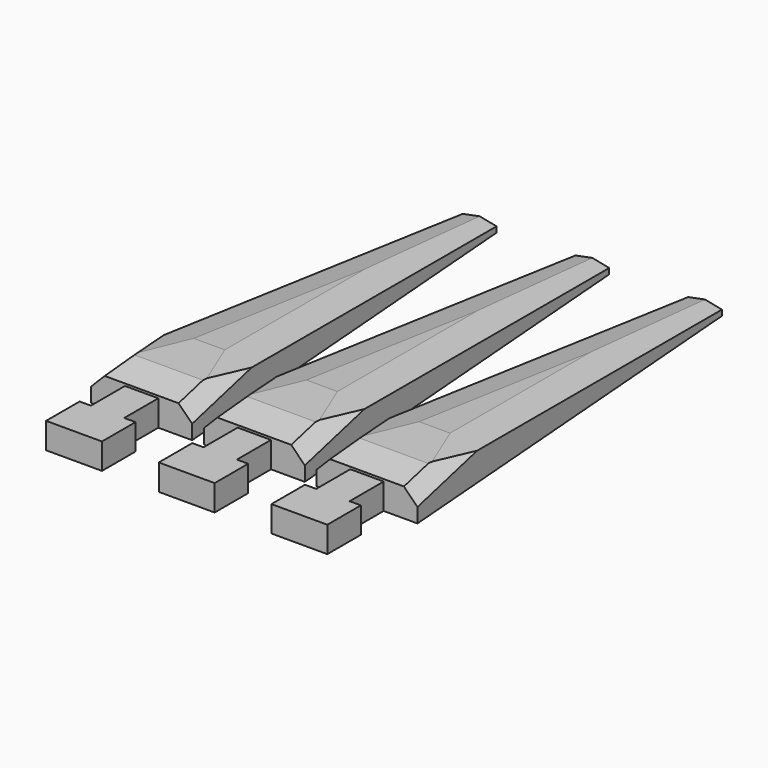
from build123d import *

# Parameters (mm, degrees)
F0_W        = 1.8796
F0_H        = 4.8006
F1_DEPTH    = 2.921
F2_DEPTH    = 3.81
F3_SIZE2    = 0.635
F3_SIZE     = 3.81
F4_SIZE2    = 2.54
F4_SIZE     = 38.1
F5_C1_SIZE  = 1.524
F5_C2_SIZE  = 1.524
F6_T1_DEPTH = 68.7483061083
F6_T3_DEPTH = 68.7483061083


# Not quite as in the source:
# - a fillet or chamfer that OpenCascade refuses, or shapes differently, is made with other operations: its cross-section is extruded or revolved along the edge and cut away or added


with BuildPart() as f1:
    # F0 (on Top) → F1 (new body)
    with BuildSketch(Plane.XY):
        Polygon((3.1496, -2.3622), (3.1496, 2.3622), (1.8796, 2.3622), (0, 2.3622), (-1.8796, 2.3622), (-3.1496, 2.3622), (-3.1496, -2.3622), align=None)
        with Locations((0.9398, 4.7625)):
            Rectangle(F0_W, F0_H)
        with Locations((-0.9398, 4.7625)):
            Rectangle(F0_W, F0_H)
    extrude(amount=F1_DEPTH)

    # F0 (on Top) → F2 (join)
    with BuildSketch(Plane.XY):
        Polygon((0, 7.1628), (1.8796, 7.1628), (5.6896, 7.1628), (1.905, 54.7878), (0, 54.7878), (-1.905, 54.7878), (-5.6896, 7.1628), (-1.8796, 7.1628), align=None)
    extrude(amount=F2_DEPTH)

    # F3
    f3_edges = [f1.edges().sort_by_distance(p)[0] for p in [
        (0, 7.1628, 3.81),
    ]]
    f3_side = f1.faces().sort_by_distance((0, 27.019823, 3.81))[0]
    chamfer(f3_edges, length=F3_SIZE, length2=F3_SIZE2, reference=f3_side)

    # F4
    f4_edges = [f1.edges().sort_by_distance(p)[0] for p in [
        (0, 54.7878, 3.81),
    ]]
    f4_side = f1.faces().sort_by_distance((0, 29.393374, 3.81))[0]
    chamfer(f4_edges, length=F4_SIZE, length2=F4_SIZE2, reference=f4_side)

    # F5: chamfer of 1.524 on 2 edges, made by hand

    # F5_c1
    f5_c1_edges = [f1.edges().sort_by_distance(p)[0] for p in [
        (5.538216, 9.0678, 3.4925),
    ]]
    chamfer(f5_c1_edges, length=F5_C1_SIZE)

    # F5_c2
    f5_c2_edges = [f1.edges().sort_by_distance(p)[0] for p in [
        (-5.538216, 9.0678, 3.4925),
    ]]
    chamfer(f5_c2_edges, length=F5_C2_SIZE)

    # F6: chamfer of 0.635 x 3.175 on 2 edges, made by hand

    # F6_s2 → F6_t1 (cut)
    with BuildSketch(Plane(origin=(-0.4931150258, -6.2053065323, 0.4136871022), x_dir=(-0.9968574007, 0.0792169348, 0), z_dir=(0.0790425792, 0.9946633283, -0.0663108886))):
        Polygon((3.0641790074, 4.8955388795), (6.2391349272, 4.2438084325), (6.2391349272, 4.8788084325), align=None)
    extrude(amount=F6_T1_DEPTH, mode=Mode.SUBTRACT)

    # F6_s4 → F6_t3 (cut)
    with BuildSketch(Plane(origin=(0.4931150258, -6.2053065323, 0.4136871022), x_dir=(-0.9968574007, -0.0792169348, 0), z_dir=(-0.0790425792, 0.9946633283, -0.0663108886))):
        Polygon((-3.0641790074, 4.8955388795), (-6.2391349272, 4.2438084325), (-6.2391349272, 4.8788084325), align=None)
    extrude(amount=F6_T3_DEPTH, mode=Mode.SUBTRACT)


with BuildPart() as f7_1:
    # F7: copy of F1
    add(f1.part.moved(Location((12.7, 0, 0))))


with BuildPart() as f8_1:
    # F8: copy of F1
    add(f1.part.moved(Location((-12.7, 0, 0))))


solid = Compound([f1.part, f7_1.part, f8_1.part])
